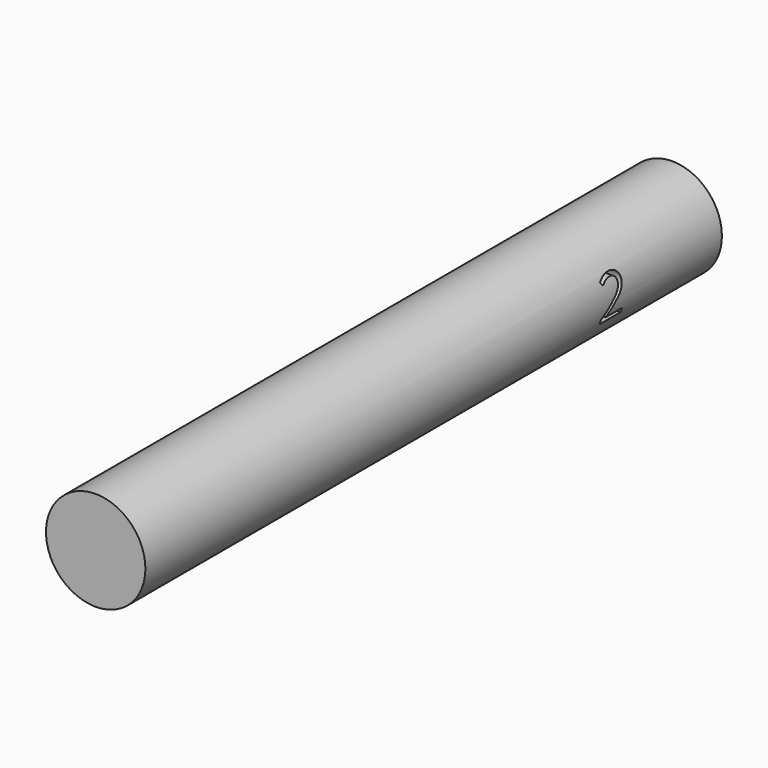
from build123d import *

# Parameters (mm, degrees)
F0_R         = 31.7070359
F1_DEPTH     = 459.74
F2_TEXT_SIZE = 36.1966357256
F3_DEPTH     = 701.04


# Not quite as in the source:
# - Text() gives the source's letters only with a copy of the font that has no kerning and outlines rounded to 1/6400 em; it was checked with that copy


with BuildPart() as f1:
    # F0 (on Front) → F1 (new body)
    with BuildSketch(Plane.XZ):
        Circle(F0_R)
    extrude(amount=F1_DEPTH)

    # F2 (on Right) → F3 (cut)
    with BuildSketch(Plane.YZ):
        with Locations((-96.6935157776, -11.8242343888)):
            Text('2', F2_TEXT_SIZE, font='Open Sans', text_align=(TextAlign.LEFT, TextAlign.BOTTOM))
    extrude(amount=F3_DEPTH, mode=Mode.SUBTRACT)


solid = f1.part
